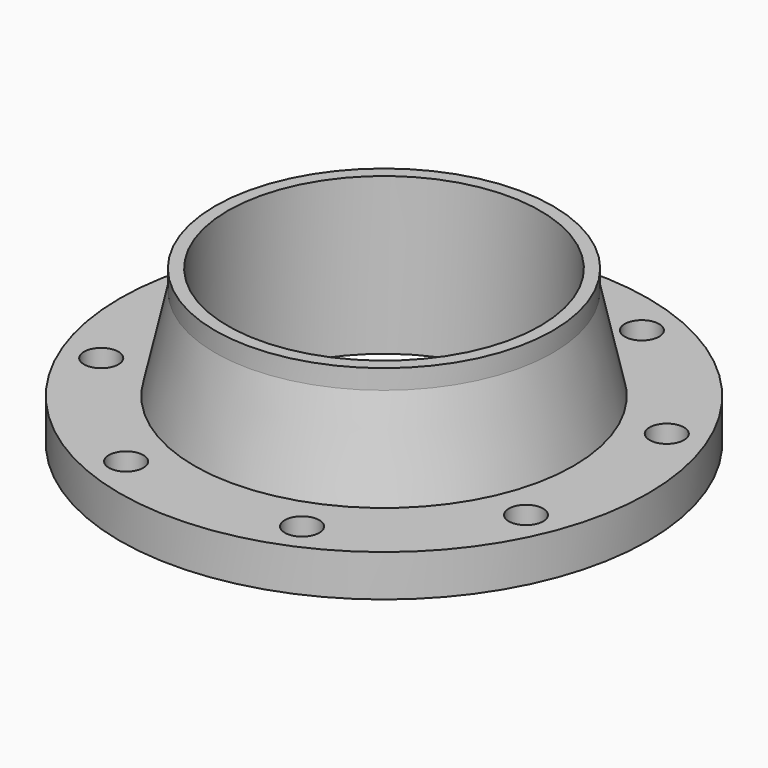
from build123d import *

# Parameters (mm, degrees)
F1_R            = 11.176
F3_DEPTH        = 101.601
F3_COPIES_COUNT = 8


# Not quite as in the source:
# - a pattern or mirror of a feature is missing from the dataset's text; its kind, count and spacing are read off the source's solid


with BuildPart() as f2:
    # F0 (on Front) → F2 (revolve)
    with BuildSketch(Plane.XZ):
        Polygon((101.346, 101.6), (101.346, 0), (135.001, 0), (135.001, 1.5875), (171.45, 1.5875), (171.45, 28.702), (123.063, 28.702), (109.601, 88.9), (109.601, 101.6), align=None)
    revolve(axis=Axis((0, 0, 50.8), (0, 0, 1)))

    # F1 (on Top) → F3 (cut, through all)
    with BuildSketch(Plane.XY):
        with Locations((137.865923239, 57.1059351947)):
            Circle(F1_R)
    f3 = extrude(amount=F3_DEPTH, mode=Mode.SUBTRACT)

    # F3_copies: F3 ×8 about axis
    f3_copies_axis = Axis((0, 0, 0), (0, 0, 1))
    for i in range(1, F3_COPIES_COUNT):
        add(f3.rotate(f3_copies_axis, i * 360 / F3_COPIES_COUNT), mode=Mode.SUBTRACT)


solid = f2.part
